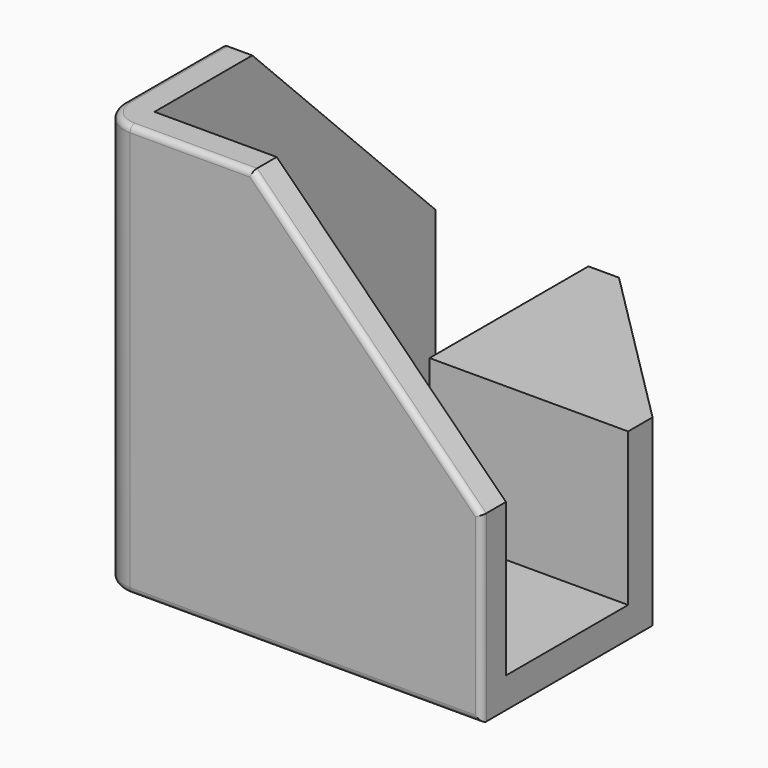
from build123d import *

# Parameters (mm, degrees)
F1_DEPTH     = 24
F3_DEPTH     = 20
F4_DEPTH     = 30
F6_DEPTH     = 25
F8_DEPTH     = 25
F9_R         = 0.8
F10_T1_DEPTH = 54
F10_T4_ANGLE = 90
F10_T6_ANGLE = 90


# Not quite as in the source:
# - a fillet or chamfer that OpenCascade refuses, or shapes differently, is made with other operations: its cross-section is extruded or revolved along the edge and cut away or added


with BuildPart() as f1:
    # F0 (on Top) → F1 (new body)
    with BuildSketch(Plane.XY):
        Polygon((-36.005956176, 35.1195232451), (-64.005956176, 35.1195232451), (-64.005956176, -14.8804767549), (-14.005956176, -14.8804767549), (-14.005956176, 13.1195232451), align=None)
    extrude(amount=F1_DEPTH)

    # F2 (on face) → F3 (cut)
    with BuildSketch(Plane.XY.offset(24)):
        Polygon((-40.005956176, 35.1195232451), (-60.005956176, 35.1195232451), (-60.005956176, -10.8804767549), (-14.005956176, -10.8804767549), (-14.005956176, 9.1195232451), (-40.005956176, 9.1195232451), align=None)
    extrude(amount=-F3_DEPTH, mode=Mode.SUBTRACT)

    # F4 (add): a face of the model
    f4_faces = [f1.faces().sort_by_distance(p)[0] for p in [
        (-60.7130629571, 12.1195232451, 24),
    ]]
    extrude(f4_faces, amount=F4_DEPTH)

    # F5 (on face) → F6 (cut)
    with BuildSketch(Plane.XZ.offset(14.8804767549)):
        Polygon((-14.005956176, 24), (-14.005956176, 54), (-44.005956176, 54), align=None)
    extrude(amount=-F6_DEPTH, mode=Mode.SUBTRACT)

    # F7 (on face) → F8 (cut)
    with BuildSketch(Plane(origin=(-64.005956176, 0, 0), x_dir=(0, -1, 0), z_dir=(-1, 0, 0))):
        Polygon((-5.1195232451, 54), (-35.1195232451, 54), (-35.1195232451, 24), align=None)
    extrude(amount=-F8_DEPTH, mode=Mode.SUBTRACT)

    # F9
    f9_edges = [f1.edges().sort_by_distance(p)[0] for p in [
        (-64.005956, -4.880477, 54),
        (-54.005956, -14.880477, 54),
        (-64.005956, 20.119523, 39),
        (-29.005956, -14.880477, 39),
        (-64.005956, 35.119523, 12),
        (-14.005956, -14.880477, 12),
        (-64.005956, 10.119523, 0),
        (-39.005956, -14.880477, 0),
    ]]
    fillet(f9_edges, radius=F9_R)

    # F10: fillet of radius 4 on 1 edges, made by hand

    # F10_s2 → F10_t1 (cut)
    with BuildSketch(Plane.XY):
        with BuildLine():
            ThreePointArc((-64.005956176, -10.8804767549), (-62.8343833007, -13.7089038797), (-60.005956176, -14.8804767549))
            Line((-60.005956176, -14.8804767549), (-64.005956176, -14.8804767549))
            Line((-64.005956176, -14.8804767549), (-64.005956176, -10.8804767549))
        make_face()
    extrude(amount=F10_T1_DEPTH, mode=Mode.SUBTRACT)

    # F10_s3 → F10_t4 (revolve, cut)
    with BuildSketch(Plane.YZ.offset(-60.005956176)):
        with BuildLine():
            ThreePointArc((-14.0804767549, 0), (-14.6461621799, 0.2343145751), (-14.8804767549, 0.8))
            Line((-14.8804767549, 0.8), (-14.8804767549, 0))
            Line((-14.8804767549, 0), (-14.0804767549, 0))
        make_face()
    revolve(axis=Axis((-60.005956176, -10.8804767549, 0), (0, 0, -1)), revolution_arc=F10_T4_ANGLE, mode=Mode.SUBTRACT)

    # F10_s5 → F10_t6 (revolve, cut)
    with BuildSketch(Plane.XZ.offset(10.8804767549)):
        with BuildLine():
            ThreePointArc((-63.205956176, 54), (-63.7716416009, 53.7656854249), (-64.005956176, 53.2))
            Line((-64.005956176, 53.2), (-64.005956176, 54))
            Line((-64.005956176, 54), (-63.205956176, 54))
        make_face()
    revolve(axis=Axis((-60.005956176, -10.8804767549, 54), (0, 0, 1)), revolution_arc=F10_T6_ANGLE, mode=Mode.SUBTRACT)


solid = f1.part
